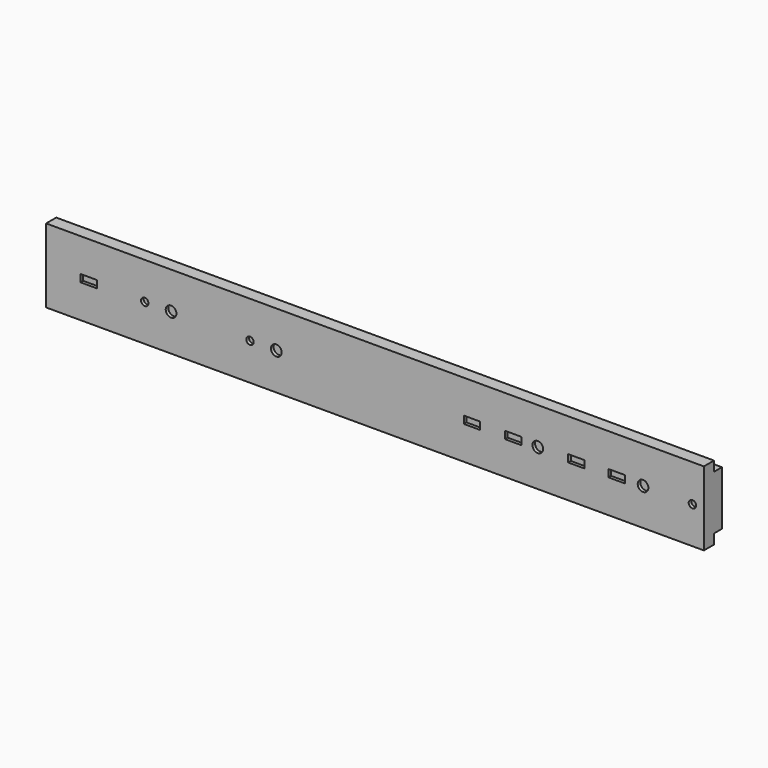
from build123d import *

# Parameters (mm, degrees)
F0_W         = 400
F0_H         = 45
F1_DEPTH     = 13.7
F2_R         = 2.25
F2_R_2       = 3.25
F2_W         = 10
F2_H         = 4.5
F3_DEPTH     = 2
F4_R         = 2.25
F4_W         = 4.5
F4_H         = 10
F4_W_2       = 10
F4_H_2       = 4.5
F5_DEPTH     = 2
F6_W         = 400
F6_H         = 6
F7_DEPTH     = 6
F8_T1_DEPTH  = 7.875
F9_TEXT_SIZE = 11.7373348783
F10_DEPTH    = 2


# Not quite as in the source:
# - a fillet or chamfer that OpenCascade refuses, or shapes differently, is made with other operations: its cross-section is extruded or revolved along the edge and cut away or added
# - Text() gives the source's letters only with a copy of the font that has no kerning and outlines rounded to 1/6400 em; it was checked with that copy


with BuildPart() as f1:
    # F0 (on Front) → F1 (new body)
    with BuildSketch(Plane.XZ):
        Rectangle(F0_W, F0_H)
    extrude(amount=F1_DEPTH)

    # F2 (on face) → F3 (cut)
    with BuildSketch(Plane.XZ.offset(13.7)):
        with Locations((-140, 0)):
            Circle(F2_R)
        with Locations((-124, 0)):
            Circle(F2_R_2)
        with Locations((-76, 0)):
            Circle(F2_R)
        with Locations((-60, 0)):
            Circle(F2_R_2)
        with Locations((-174, 0)):
            Rectangle(F2_W, F2_H)
        with Locations((59, 0)):
            Rectangle(F2_W, F2_H)
        with Locations((84, 0)):
            Rectangle(F2_W, F2_H)
        with Locations((99, 0)):
            Circle(F2_R_2)
        with Locations((122.5, 0)):
            Rectangle(F2_W, F2_H)
        with Locations((147, 0)):
            Rectangle(F2_W, F2_H)
        with Locations((163, 0)):
            Circle(F2_R_2)
        with Locations((193, 0)):
            Circle(F2_R)
    extrude(amount=-F3_DEPTH, mode=Mode.SUBTRACT)

    # F4 (on face) → F5 (cut)
    with BuildSketch(Plane(origin=(0, 0, 0), x_dir=(-1, 0, 0), z_dir=(0, 1, 0))):
        Polygon((195, 10), (195, -10), (200, -14), (200, 14), align=None)
        with Locations((181, 0)):
            Circle(F4_R)
        with Locations((171.5, 0)):
            Rectangle(F4_W, F4_H)
        with Locations((156, 0)):
            Rectangle(F4_W_2, F4_H_2)
        with Locations((90, 0)):
            Circle(F4_R)
        with Locations((-11.5, 0)):
            Circle(F4_R)
        with Locations((-21, 0)):
            Rectangle(F4_W, F4_H)
        with Locations((-36.5, 0)):
            Rectangle(F4_W_2, F4_H_2)
        with Locations((-139, 0)):
            Circle(F4_R)
        with Locations((-148.5, 0)):
            Rectangle(F4_W, F4_H)
        with Locations((-164, 0)):
            Rectangle(F4_W_2, F4_H_2)
    extrude(amount=-F5_DEPTH, mode=Mode.SUBTRACT)

    # F6 (on face) → F7 (cut)
    with BuildSketch(Plane(origin=(0, 0, 0), x_dir=(-1, 0, 0), z_dir=(0, 1, 0))):
        with Locations((0, -19.5)):
            Rectangle(F6_W, F6_H)
        with Locations((0, 19.5)):
            Rectangle(F6_W, F6_H)
    extrude(amount=-F7_DEPTH, mode=Mode.SUBTRACT)

    # F8: fillet of radius 2.35 on 8 edges, made by hand

    # F8_s2 → F8_t1 (join)
    with BuildSketch(Plane.XZ):
        with BuildLine():
            ThreePointArc((-171.4, 5), (-173.0617009358, 4.3117009358), (-173.75, 2.65))
            Line((-173.75, 2.65), (-173.75, 5))
            Line((-173.75, 5), (-171.4, 5))
        make_face()
        with BuildLine():
            ThreePointArc((-173.75, -2.65), (-173.0617009358, -4.3117009358), (-171.4, -5))
            Line((-171.4, -5), (-173.75, -5))
            Line((-173.75, -5), (-173.75, -2.65))
        make_face()
        with BuildLine():
            ThreePointArc((-169.25, -2.65), (-169.9382990642, -4.3117009358), (-171.6, -5))
            Line((-171.6, -5), (-169.25, -5))
            Line((-169.25, -5), (-169.25, -2.65))
        make_face()
        with BuildLine():
            ThreePointArc((-171.6, 5), (-169.9382990642, 4.3117009358), (-169.25, 2.65))
            Line((-169.25, 2.65), (-169.25, 5))
            Line((-169.25, 5), (-171.6, 5))
        make_face()
        with BuildLine():
            ThreePointArc((-153.35, 2.25), (-151.6882990642, 1.5617009358), (-151, -0.1))
            Line((-151, -0.1), (-151, 2.25))
            Line((-151, 2.25), (-153.35, 2.25))
        make_face()
        with BuildLine():
            ThreePointArc((-161, 0.1), (-160.3117009358, -1.5617009358), (-158.65, -2.25))
            Line((-158.65, -2.25), (-161, -2.25))
            Line((-161, -2.25), (-161, 0.1))
        make_face()
        with BuildLine():
            ThreePointArc((-161, -0.1), (-160.3117009358, 1.5617009358), (-158.65, 2.25))
            Line((-158.65, 2.25), (-161, 2.25))
            Line((-161, 2.25), (-161, -0.1))
        make_face()
        with BuildLine():
            ThreePointArc((-153.35, -2.25), (-151.6882990642, -1.5617009358), (-151, 0.1))
            Line((-151, 0.1), (-151, -2.25))
            Line((-151, -2.25), (-153.35, -2.25))
        make_face()
    extrude(amount=F8_T1_DEPTH)

    # F9 (on face) → F10 (cut)
    with BuildSketch(Plane(origin=(0, 0, 0), x_dir=(-1, 0, 0), z_dir=(0, 1, 0))):
        with Locations((48.1507889926, -14.2392776906)):
            Text('drawer side fixed end', F9_TEXT_SIZE, font='Open Sans', text_align=(TextAlign.LEFT, TextAlign.BOTTOM))
    extrude(amount=-F10_DEPTH, mode=Mode.SUBTRACT)


solid = f1.part
